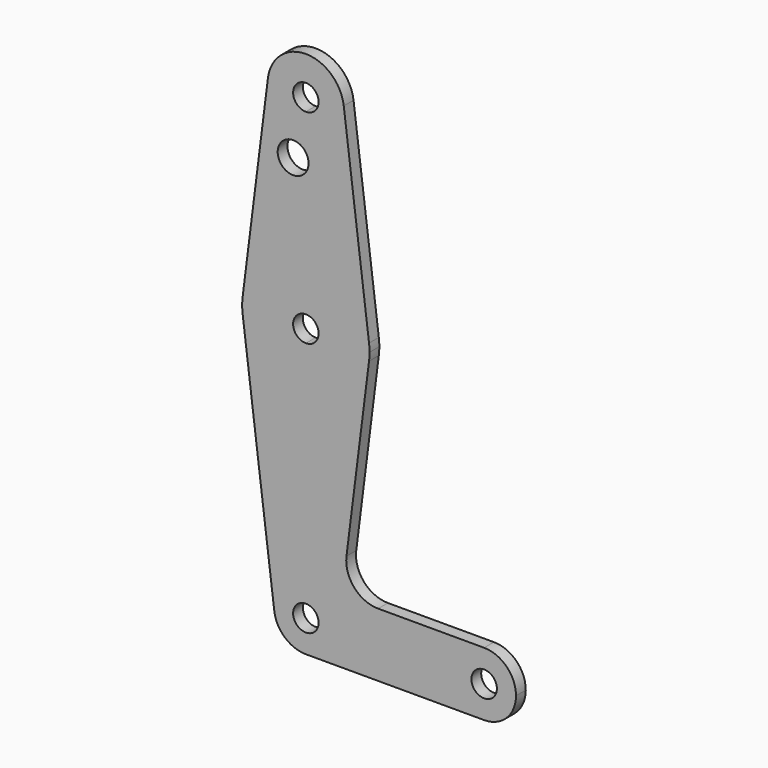
from build123d import *

# Parameters (mm, degrees)
F1_DEPTH = 3.048


with BuildPart() as f1:
    # F0 (on Front) → F1 (new body)
    with BuildSketch(Plane.XZ):
        with BuildLine():
            ThreePointArc((9.4502929642, 115.490625), (0, 123.825), (-9.4502929642, 115.490625))
            ThreePointArc((-9.4502929642, 115.490625), (-7.14375, 107.9998046905), (0, 104.775))
            ThreePointArc((0, 104.775), (6.7351920908, 107.5648079092), (9.525, 114.3))
            ThreePointArc((9.525, 114.3), (9.5063048942, 114.896483242), (9.4502929642, 115.490625))
        make_face()
        with BuildLine():
            ThreePointArc((3.175, 114.3), (2.2450640303, 112.0549359697), (0, 111.125))
            ThreePointArc((0, 111.125), (-2.2450640303, 116.5450640303), (3.175, 114.3))
        make_face(mode=Mode.SUBTRACT)
        with BuildLine():
            Line((-9.4502929642, 115.490625), (-15.7504882737, 65.484375))
            ThreePointArc((-15.7504882737, 65.484375), (-10.5003255158, 75.40625), (0, 79.375))
            Line((0, 79.375), (0, 97.8521401046))
            ThreePointArc((0, 97.8521401046), (-7.0224425673, 100.0252), (0, 102.1982598954))
            Line((0, 102.1982598954), (0, 104.775))
            ThreePointArc((0, 104.775), (-7.14375, 107.9998046905), (-9.4502929642, 115.490625))
        make_face()
        with BuildLine():
            Line((0, 97.8521401046), (0, 79.375))
            ThreePointArc((0, 79.375), (10.5003255158, 75.40625), (15.7504882737, 65.484375))
            Line((15.7504882737, 65.484375), (9.4502929642, 115.490625))
            ThreePointArc((9.4502929642, 115.490625), (9.5063048942, 114.896483242), (9.525, 114.3))
            ThreePointArc((9.525, 114.3), (6.7351920908, 107.5648079092), (0, 104.775))
            Line((0, 104.775), (0, 102.1982598954))
            ThreePointArc((0, 102.1982598954), (0.5004893865, 101.1625618944), (0.6724425673, 100.0252))
            ThreePointArc((0.6724425673, 100.0252), (0.5004893865, 98.8878381056), (0, 97.8521401046))
        make_face()
        with BuildLine():
            Line((0, 47.625), (0, 7.9375))
            ThreePointArc((0, 7.9375), (5.6126600757, 5.6126600757), (7.9375, 0))
            Line((7.9375, 0), (36.5125, 0))
            ThreePointArc((36.5125, 0), (38.8373399243, 5.6126600757), (44.45, 7.9375))
            Line((44.45, 7.9375), (18.0149584735, 7.9375))
            ThreePointArc((18.0149584735, 7.9375), (12.0523084735, 10.6291369817), (10.127113946, 16.881475))
            Line((10.127113946, 16.881475), (15.7504882737, 61.515625))
            ThreePointArc((15.7504882737, 61.515625), (10.5003255158, 51.59375), (0, 47.625))
        make_face()
        with BuildLine():
            Line((0, 60.325), (0, 47.625))
            ThreePointArc((0, 47.625), (10.5003255158, 51.59375), (15.7504882737, 61.515625))
            ThreePointArc((15.7504882737, 61.515625), (15.8438414904, 62.5058612634), (15.875, 63.5))
            ThreePointArc((15.875, 63.5), (15.8438414904, 64.4941387366), (15.7504882737, 65.484375))
            ThreePointArc((15.7504882737, 65.484375), (10.5003255158, 75.40625), (0, 79.375))
            Line((0, 79.375), (0, 66.675))
            ThreePointArc((0, 66.675), (2.2450640303, 65.7450640303), (3.175, 63.5))
            ThreePointArc((3.175, 63.5), (2.2450640303, 61.2549359697), (0, 60.325))
        make_face()
        with BuildLine():
            ThreePointArc((-15.7504882737, 61.515625), (-10.5003255158, 51.59375), (0, 47.625))
            Line((0, 47.625), (0, 60.325))
            ThreePointArc((0, 60.325), (-3.175, 63.5), (0, 66.675))
            Line((0, 66.675), (0, 79.375))
            ThreePointArc((0, 79.375), (-10.5003255158, 75.40625), (-15.7504882737, 65.484375))
            ThreePointArc((-15.7504882737, 65.484375), (-15.875, 63.5), (-15.7504882737, 61.515625))
        make_face()
        with BuildLine():
            ThreePointArc((-7.8752441368, -0.9921875), (-5.953125, 5.2501627579), (0, 7.9375))
            Line((0, 7.9375), (0, 47.625))
            ThreePointArc((0, 47.625), (-10.5003255158, 51.59375), (-15.7504882737, 61.515625))
            Line((-15.7504882737, 61.515625), (-7.8752441368, -0.9921875))
        make_face()
        with BuildLine():
            Line((36.5125, 0), (7.9375, 0))
            ThreePointArc((7.9375, 0), (5.6126600757, -5.6126600757), (0, -7.9375))
            Line((0, -7.9375), (44.45, -7.9375))
            ThreePointArc((44.45, -7.9375), (38.8373399243, -5.6126600757), (36.5125, 0))
        make_face()
        with BuildLine():
            ThreePointArc((44.45, 7.9375), (38.8373399243, 5.6126600757), (36.5125, 0))
            ThreePointArc((36.5125, 0), (38.8373399243, -5.6126600757), (44.45, -7.9375))
            ThreePointArc((44.45, -7.9375), (50.0626600757, -5.6126600757), (52.3875, 0))
            ThreePointArc((52.3875, 0), (50.0626600757, 5.6126600757), (44.45, 7.9375))
        make_face()
        with BuildLine():
            ThreePointArc((47.625, 0), (44.45, -3.175), (41.275, 0))
            ThreePointArc((41.275, 0), (44.45, 3.175), (47.625, 0))
        make_face(mode=Mode.SUBTRACT)
        with BuildLine():
            ThreePointArc((3.175, 0), (-2.2450640303, -2.2450640303), (0, 3.175))
            Line((0, 3.175), (0, 7.9375))
            ThreePointArc((0, 7.9375), (-5.953125, 5.2501627579), (-7.8752441368, -0.9921875))
            ThreePointArc((-7.8752441368, -0.9921875), (-5.2501627579, -5.953125), (0, -7.9375))
            ThreePointArc((0, -7.9375), (5.6126600757, -5.6126600757), (7.9375, 0))
            Line((7.9375, 0), (3.175, 0))
        make_face()
        with BuildLine():
            Line((0, 7.9375), (0, 3.175))
            ThreePointArc((0, 3.175), (2.2450640303, 2.2450640303), (3.175, 0))
            Line((3.175, 0), (7.9375, 0))
            ThreePointArc((7.9375, 0), (5.6126600757, 5.6126600757), (0, 7.9375))
        make_face()
    extrude(amount=F1_DEPTH)


solid = f1.part
